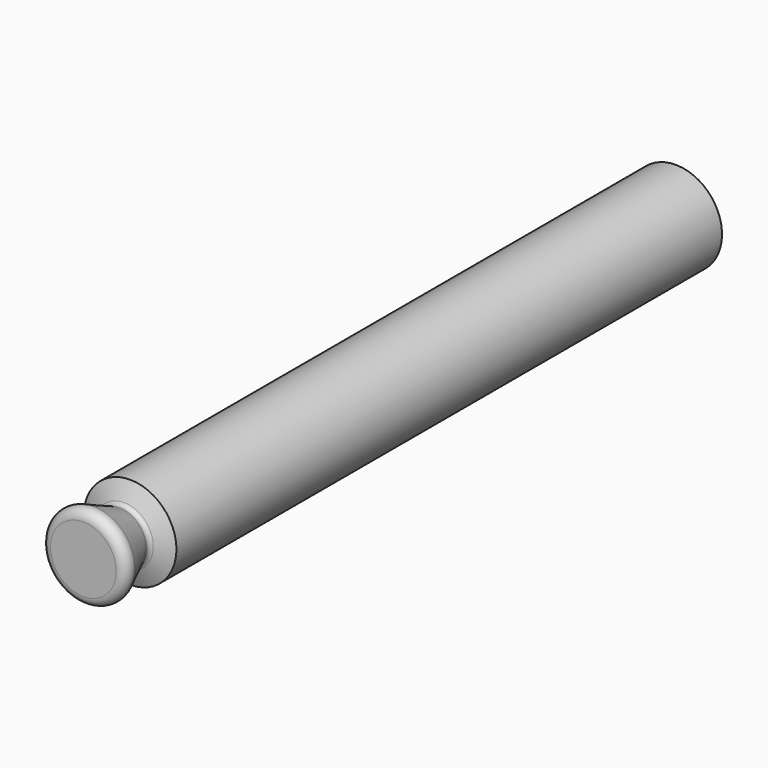
from build123d import *


# Not quite as in the source:
# - ends of sketch curves that miss each other by under 0.0002 mm in the source are joined


with BuildPart() as f2:
    # F1 (on Top) → F2 (revolve)
    with BuildSketch(Plane.XY):
        with BuildLine():
            ThreePointArc((-1.5543495265, -30.6423329465), (-1.4953949864, -31.3914475732), (-0.835025, -31.75))
            Line((-0.835025, -31.75), (1.984375, -31.75))
            Line((1.984375, -31.75), (1.984375, 31.75))
            Line((1.984375, 31.75), (-1.984375, 31.75))
            Line((-1.984375, 31.75), (-1.984375, -26.7380212))
            Line((-1.984375, -26.7380212), (-0.5228082, -27.3887438))
            ThreePointArc((-0.5228082, -27.3887438), (-0.322079197, -27.6002624898), (-0.3297130763, -27.8917673251))
            Line((-0.3297130763, -27.8917673251), (-1.5543495265, -30.6423329465))
        make_face()
    revolve(axis=Axis((1.984375, 0, 0), (0, -1, 0)))


solid = f2.part
